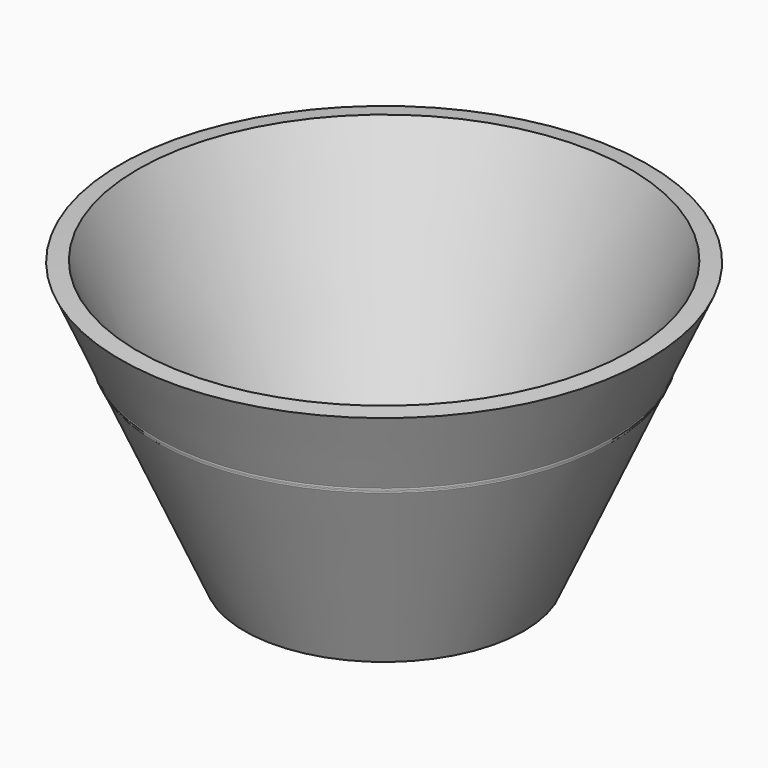
from build123d import *


# Not quite as in the source:
# - a feature names something its author has since deleted; it is built from what else it names


with BuildPart() as f1:
    # F0 (on Front) → F1 (revolve)
    with BuildSketch(Plane.XZ):
        Polygon((0, 3.0699997223), (0, 0), (25.4, 0), (41.0826989019, 35.2669842541), (41.2241344504, 35.5850420892), (41.3456860605, 35.8583852649), (41.4835813014, 36.1684817169), (47.9899980128, 50.8), (44.7618767703, 51.0962395517), (23.4053282997, 3.0699997223), align=None)
        Polygon((41.4835813014, 36.1684817169), (41.3456860605, 35.8583852649), (41.4835813014, 35.8583852649), align=None)
        Polygon((41.3456860605, 35.8583852649), (41.2241344504, 35.5850420892), (41.3456860605, 35.5850420892), align=None)
        Polygon((41.2241344504, 35.5850420892), (41.0826989019, 35.2669842541), (41.2241344504, 35.2669842541), align=None)
    revolve(axis=Axis((0, 0, 25.4), (0, 0, 1)))


solid = f1.part
